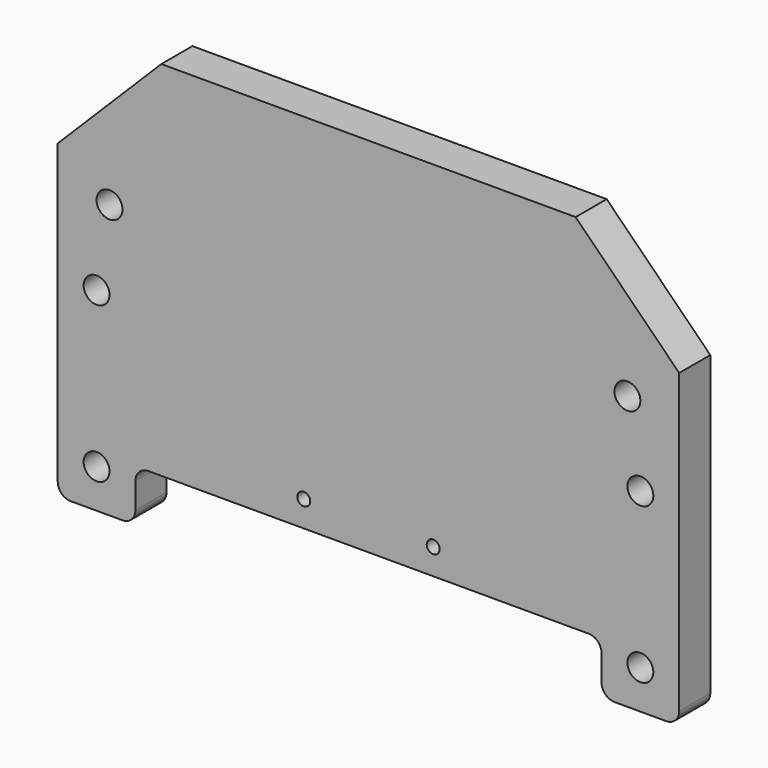
from build123d import *

# Parameters (mm, degrees)
F1_DEPTH       = 19.05
F2_R           = 6.35
F3_SIZE2       = 50.8
F3_SIZE        = 50.8
F4_R           = 3.175
F5_DEPTH       = 25.4
F6_D           = 12.7
F6_DEPTH       = 12.7
F6_TIP         = 3.8154649308
F7_D           = 9.525
F7_DEPTH       = 25.4
F7_CBORE_D     = 12.7
F7_CBORE_DEPTH = 12.7
F7_TIP         = 2.8615986981


# Not quite as in the source:
# - a feature names something its author has since deleted; it is built from what else it names


with BuildPart() as f1:
    # F0 (on Front) → F1 (new body)
    with BuildSketch(Plane.XZ):
        Polygon((-61.5315027535, 184.1499997646), (-61.5315027535, -19.0500002354), (-23.4315027535, -19.0500002354), (-23.4315027535, 6.3499997646), (205.1684972465, 6.3499997646), (205.1684972465, -19.0500002354), (243.2684972465, -19.0500002354), (243.2684972465, 184.1499997646), align=None)
    extrude(amount=F1_DEPTH)

    # F2
    f2_edges = [f1.edges().sort_by_distance(p)[0] for p in [
        (-23.431503, -9.525, 6.35),
        (-61.531503, -9.525, -19.05),
        (243.268497, -9.525, -19.05),
        (205.168497, -9.525, -19.05),
        (205.168497, -9.525, 6.35),
        (-23.431503, -9.525, -19.05),
    ]]
    fillet(f2_edges, radius=F2_R)

    # F3
    f3_edges = [f1.edges().sort_by_distance(p)[0] for p in [
        (243.268497, -9.525, 184.15),
        (-61.531503, -9.525, 184.15),
    ]]
    chamfer(f3_edges, length=F3_SIZE, length2=F3_SIZE2)

    # F4 (on face) → F5 (cut)
    with BuildSketch(Plane.XZ.offset(19.05)):
        with Locations((59.1184972465, 19.0499997646)):
            Circle(F4_R)
        with Locations((122.6184972465, 19.0499997646)):
            Circle(F4_R)
    extrude(amount=-F5_DEPTH, mode=Mode.SUBTRACT)

    # F6
    with Locations(Plane.XZ.offset(19.05)):
        with Locations((-36.1315027535, 115.1381997646), (217.8684972465, 115.1381997646)):
            Hole(F6_D / 2, depth=F6_DEPTH)
            with Locations((0, 0, -(F6_DEPTH + F6_TIP / 2))):  # 118° drill point
                Cone(0, F6_D / 2, F6_TIP, mode=Mode.SUBTRACT)

    # F7
    with Locations(Plane.XZ.offset(19.05)):
        with Locations((-42.4815027535, 76.1999997646), (-42.4815027535, -2.354e-07), (224.2184972465, -2.354e-07), (224.2184972465, 76.1999997646)):
            CounterBoreHole(F7_D / 2, F7_CBORE_D / 2, F7_CBORE_DEPTH, depth=F7_DEPTH)
            with Locations((0, 0, -(F7_DEPTH + F7_TIP / 2))):  # 118° drill point
                Cone(0, F7_D / 2, F7_TIP, mode=Mode.SUBTRACT)


solid = f1.part
